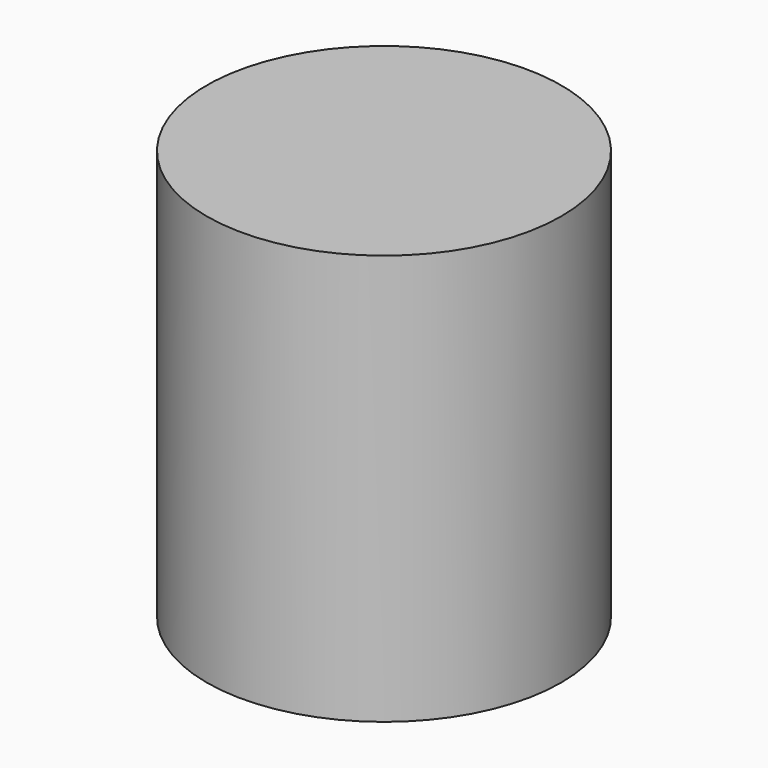
from build123d import *

# Parameters (mm, degrees)
F0_R     = 73.4453519662
F0_R_2   = 16.6359936191
F1_DEPTH = 37.0360137895
F4_R     = 73.4453519662
F4_R_2   = 16.6359936191
F4_R_3   = 15.9987703345
F2_DEPTH = 50.8


# Not quite as in the source:
# - a feature names something its author has since deleted; it is built from what else it names


with BuildPart() as f1:
    # F0 (on Top) → F1 (new body)
    with BuildSketch(Plane.XY):
        Circle(F0_R)
        Circle(F0_R_2, mode=Mode.SUBTRACT)
    extrude(amount=F1_DEPTH)

    # F4 (on face) → F2 (cut)
    with BuildSketch(Plane.XY.offset(37.0360137895)):
        Circle(F4_R)
        Circle(F4_R_2, mode=Mode.SUBTRACT)
        with Locations((31.0444459319, 42.349152267)):
            Circle(F4_R_3, mode=Mode.SUBTRACT)
    extrude(amount=-F2_DEPTH, mode=Mode.SUBTRACT)


solid = f1.part
